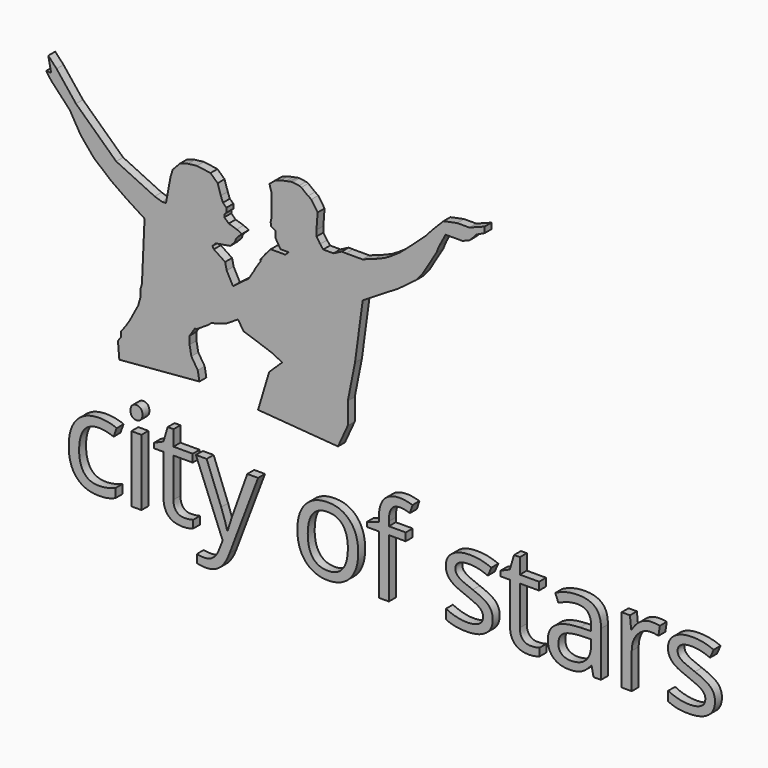
from build123d import *

# Parameters (mm, degrees)
F1_DEPTH     = 25.4
F2_TEXT_SIZE = 362.9590902064
F3_DEPTH     = 25.4


# Not quite as in the source:
# - Text() gives the source's letters only with a copy of the font that has no kerning and outlines rounded to 1/6400 em; it was checked with that copy


with BuildPart() as f1:
    # F0 (on Front) → F1 (new body)
    with BuildSketch(Plane.XZ):
        Polygon((-79.3035775423, -173.4067052603), (-24.6085301042, -208.5677981377), (-32.240152359, -379.8480331898), (-36.4694185555, -393.8038945198), (-37.1743030846, -417.2298014164), (-43.518204242, -440.1572942734), (-46.3377423584, -444.6431100368), (-67.4840435386, -484.5170080662), (-79.4669762254, -503.4571290016), (-93.5645326972, -521.8988060951), (-93.5645326972, -536.8514657021), (-102.5362057216, -549.1262749249), (-98.4986051917, -596.6623425484), (136.2256407738, -576.725423336), (131.2856779058, -549.1262749249), (112.683698535, -519.3877220154), (107.2422415018, -491.0764992237), (107.2422415018, -467.9507017136), (123.2143044472, -443.7492787838), (126.2566447258, -444.8249042034), (135.692484163, -439.0053596454), (158.200904727, -424.9259531498), (171.1307168007, -414.7075712681), (213.5638495253, -402.083412889), (249.5289232484, -379.5866370201), (265.4423117638, -405.0270020962), (308.7952435017, -419.547855854), (350.3066897392, -434.0687096119), (378.7682652473, -448.5895633698), (340.739428997, -485.198199749), (308.0345988274, -593.7981009483), (542.2924160957, -612.0836138725), (571.141064167, -548.6221313477), (571.141064167, -485.198199749), (592.0355916023, -379.5866370201), (614.7839690883, -211.6542429741), (631.5031051636, -201.1961340904), (651.6237854958, -188.6103004217), (719.7244763374, -147.0223218203), (770.800113678, -108.7176129222), (790.1468873024, -85.7347846031), (830.3883075714, -18.9751479775), (838.9008641243, 1.8188380636), (849.7350811958, 22.0656152815), (857.473731041, 36.8402861059), (907.001554966, 36.8402861059), (927.1222352982, 44.5012301207), (938.7302994728, 55.9926442802), (947.242975235, 66.3896352053), (972.0068573952, 77.8810530901), (972.0068573952, 94.8445647955), (927.1222352982, 77.8810530901), (891.5241360664, 77.8810530901), (851.2828350067, 69.6728974581), (819.5539116859, 37.3874977231), (797.8855371475, 13.3102545515), (742.1667575836, -37.0330810547), (723.5938310623, -52.9021732509), (701.1516094208, -68.2240575552), (680.2569627762, -80.8098912239), (648.5282182693, -93.9429327846), (613.7040257454, -106.1101257801), (565.6846761703, -106.1101257801), (553.4415245056, -105.7166159153), (543.1461334229, -111.0290065408), (529.233455658, -118.1121841073), (498.9038109779, -118.1121841073), (489.9997413158, -106.8971455097), (479.1355133057, -91.1520197988), (479.1355133057, -74.1451233625), (482.5873076916, -27.7699995786), (464.1776680946, -0.1076484041), (454.6852111816, 5.5875419639), (434.8373413086, 21.2493147701), (428.2213449478, 23.6901100725), (409.2364311218, 26.1309053749), (404.9216508865, 26.1309053749), (400.6069302559, 25.5207084119), (389.6761834621, 22.8765122592), (375.0060200691, 20.2323179692), (360.0482344627, 14.9439256638), (350.3066897392, 7.7054896392), (341.3700461388, 0), (346.9874858856, -18.5190439224), (346.9874858856, -34.0009965003), (346.9874858856, -61.1730478704), (346.9874858856, -87.8039970994), (344.9541926384, -97.734183073), (346.3491797447, -108.5671186447), (352.7324795723, -111.2753450871), (358.4775328636, -114.4349500537), (359.7542047501, -118.9486756921), (359.7542047501, -134.7467005253), (373.7976253033, -158.0604255888), (397.4163176983, -158.0604255888), (388.5599076748, -167.5122231245), (344.9541926384, -167.5122231245), (329.1190564632, -185.3906065226), (324.0109682083, -192.5419569016), (321.9677209854, -195.0960159302), (318.3920383453, -199.6933221817), (317.3704147339, -203.2689899206), (314.8163557053, -203.2689899206), (314.8163557053, -209.909543395), (311.7514848709, -213.485211134), (309.1974556446, -217.5717055798), (307.1541786194, -220.6365615129), (303.5784959793, -226.2554913759), (300.0028133392, -231.8744063377), (296.9379723072, -238.0041331053), (280.5920243263, -264.0554904938), (234.6190363169, -298.7906336784), (216.2298411131, -264.5663022995), (211.6325348616, -243.6230778694), (178.4298270941, -221.6582149267), (174.4129441891, -214.5398852047), (183.5379451513, -204.801440239), (226.7340889608, -197.248276064), (240.2379661798, -182.8365772963), (243.4928066489, -172.6696509493), (251.0000917975, -164.6576755463), (260.6759963306, -155.5950165236), (245.6040097831, -148.4257727861), (222.0448090283, -141.1142868487), (209.3310866398, -129.2014271021), (209.3310866398, -120.9601559247), (215.2573075918, -115.4095306993), (215.2573075918, -102.5525274424), (204.9919962883, -92.9338485003), (198.8622695208, -76.6482725739), (189.5784418525, -47.6012449429), (168.7244176865, -28.0608572066), (128.8811713457, -22.6262547076), (102.7861461043, -25.6484653801), (78.6720184755, -33.2159568705), (58.0610444081, -55.2125393891), (51.4085665345, -76.6482725739), (38.1863899529, -148.4257727861), (26.8531031907, -148.4257727861), (4.9420828, -141.6257917881), (-107.713250595, -88.0393889015), (-131.0415396982, -66.180595094), (-177.5238960981, -22.6262547076), (-225.5014777184, 22.3291236907), (-282.3837168668, 94.1865176048), (-306.7233860493, 120.1731860638), (-298.412322998, 78.6177963018), (-313.1455779076, 78.6177963018), (-298.0837523937, 58.3961047232), (-243.3887124062, 0), (-212.1344059706, -53.5985082388), (-173.0665117502, -100.4799753428), (-123.5805153847, -142.1523839235), align=None)
    extrude(amount=F1_DEPTH)


with BuildPart() as f3:
    # F2 (on Front) → F3 (new body)
    with BuildSketch(Plane.XZ):
        with Locations((-267.1485841274, -963.616669178)):
            Text('city of stars', F2_TEXT_SIZE, font='Open Sans', text_align=(TextAlign.LEFT, TextAlign.BOTTOM))
    extrude(amount=F3_DEPTH)


solid = Compound([f1.part, f3.part])
